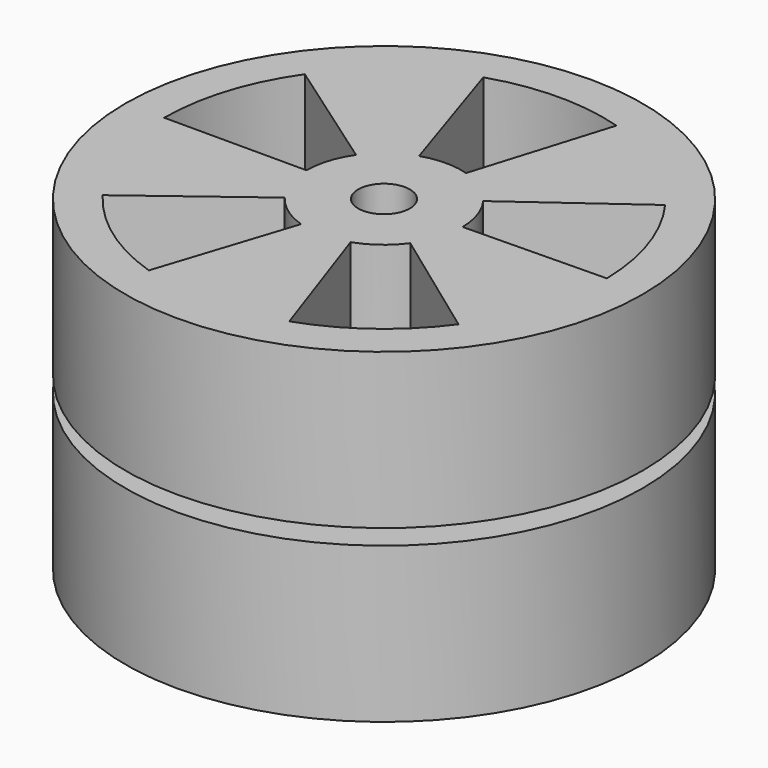
from build123d import *

# Parameters (mm, degrees)
F0_R     = 10
F1_DEPTH = 6
F2_R     = 2.5
F3_DEPTH = 0.6
F4_R     = 10
F5_DEPTH = 6
F6_R     = 1
F7_DEPTH = 25
F9_DEPTH = 12.601


with BuildPart() as f1:
    # F0 (on Top) → F1 (new body)
    with BuildSketch(Plane.XY):
        Circle(F0_R)
    extrude(amount=F1_DEPTH)

    # F2 (on face) → F3 (join)
    with BuildSketch(Plane.XY.offset(6)):
        Circle(F2_R)
    extrude(amount=F3_DEPTH)


with BuildPart() as f5:
    # F4 (on face) → F5 (new body)
    with BuildSketch(Plane.XY.offset(6.6)):
        Circle(F4_R)
    extrude(amount=F5_DEPTH)


with BuildPart() as f7_tool:
    # F6 (on face) → F7 (new body)
    with BuildSketch(Plane.XY.offset(12.6)):
        Circle(F6_R)
    extrude(amount=-F7_DEPTH)


with BuildPart() as f1_1:
    add(f1.part)

    # F7: cut by f7_tool
    add(f7_tool.part, mode=Mode.SUBTRACT)


with BuildPart() as f5_1:
    add(f5.part)

    # F7: cut by f7_tool
    add(f7_tool.part, mode=Mode.SUBTRACT)

    # F8 (on face) → F9 (cut, through all)
    with BuildSketch(Plane.XY.offset(12.6)):
        with BuildLine():
            Line((-8.5, 0), (-3, 0))
            ThreePointArc((-3, 0), (-2.8611508522, 0.9021173985), (-2.4574561329, 1.7207293091))
            Line((-2.4574561329, 1.7207293091), (-6.9627923765, 4.875399709))
            ThreePointArc((-6.9627923765, 4.875399709), (-8.1065940814, 2.5559992958), (-8.5, 0))
        make_face()
        with BuildLine():
            Line((-2.3959065301, -1.8054450695), (-6.7884018354, -5.1154276968))
            ThreePointArc((-6.7884018354, -5.1154276968), (-4.9359751235, -6.919981906), (-2.6266444522, -8.0839803885))
            Line((-2.6266444522, -8.0839803885), (-0.9270509831, -2.8531695489))
            ThreePointArc((-0.9270509831, -2.8531695489), (-1.7421088671, -2.4423465551), (-2.3959065301, -1.8054450695))
        make_face()
        with BuildLine():
            Line((0.9767044634, -2.8365557268), (2.7673293129, -8.0369078926))
            ThreePointArc((2.7673293129, -8.0369078926), (5.0559936874, -6.8327833152), (6.8766444522, -4.9961746445))
            Line((6.8766444522, -4.9961746445), (2.4270509831, -1.7633557569))
            ThreePointArc((2.4270509831, -1.7633557569), (1.7844683603, -2.4115705819), (0.9767044634, -2.8365557268))
        make_face()
        with BuildLine():
            Line((2.9995430855, 0.0523572193), (8.4987054088, 0.1483454547))
            ThreePointArc((8.4987054088, 0.1483454547), (8.0607510693, 2.6970895794), (6.8766444522, 4.9961746445))
            Line((6.8766444522, 4.9961746445), (2.4270509831, 1.7633557569))
            ThreePointArc((2.4270509831, 1.7633557569), (2.8449709656, 0.9519139692), (2.9995430855, 0.0523572193))
        make_face()
        with BuildLine():
            Line((0.8771151142, 2.8689142679), (2.4851594901, 8.1285904257))
            ThreePointArc((2.4851594901, 8.1285904257), (-0.0741755517, 8.499676346), (-2.6266444522, 8.0839803885))
            Line((-2.6266444522, 8.0839803885), (-0.9270509831, 2.8531695489))
            ThreePointArc((-0.9270509831, 2.8531695489), (-0.0261796065, 2.9998857692), (0.8771151142, 2.8689142679))
        make_face()
    extrude(amount=-F9_DEPTH, mode=Mode.SUBTRACT)


solid = Compound([f1_1.part, f5_1.part])
